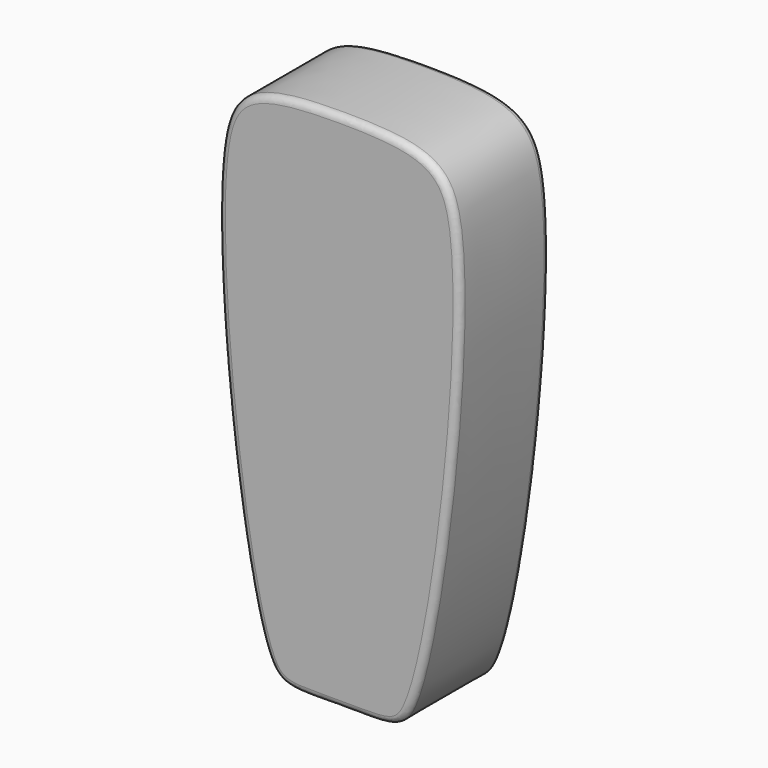
from build123d import *

# Parameters (mm, degrees)
F1_DEPTH = 25
F2_R     = 1.5


with BuildPart() as f1:
    # F0 (on Front) → F1 (new body)
    with BuildSketch(Plane.XZ):
        with BuildLine():
            add(Edge.make_bspline(
                [(0, 61.4218405223), (20.5732115106, 61.4218405223), (32.5583140399, 53.6603989504), (19.4814525281, -57.4099012602), (11.1974994913, -54.8427566432), (0, -54.8427566432)],
                knots=[0, 0, 0, 0, 0.28576922, 0.7865255737, 1, 1, 1, 1], degree=3))
            add(Edge.make_bspline(
                [(0, 61.4218405223), (-20.5732115106, 61.4218405223), (-32.5583140399, 53.6603989504), (-19.4814525281, -57.4099012602), (-11.1974994913, -54.8427566432), (0, -54.8427566432)],
                knots=[0, 0, 0, 0, 0.28576922, 0.7865255737, 1, 1, 1, 1], degree=3))
        make_face()
    extrude(amount=F1_DEPTH)

    # F2
    f2_edges = [f1.edges().sort_by_distance(p)[0] for p in [
        (-25.567038, -25, 6.077884),
        (25.567038, -25, 6.077884),
        (-25.567038, 0, 6.077884),
        (25.567038, 0, 6.077884),
    ]]
    fillet(f2_edges, radius=F2_R)


solid = f1.part
